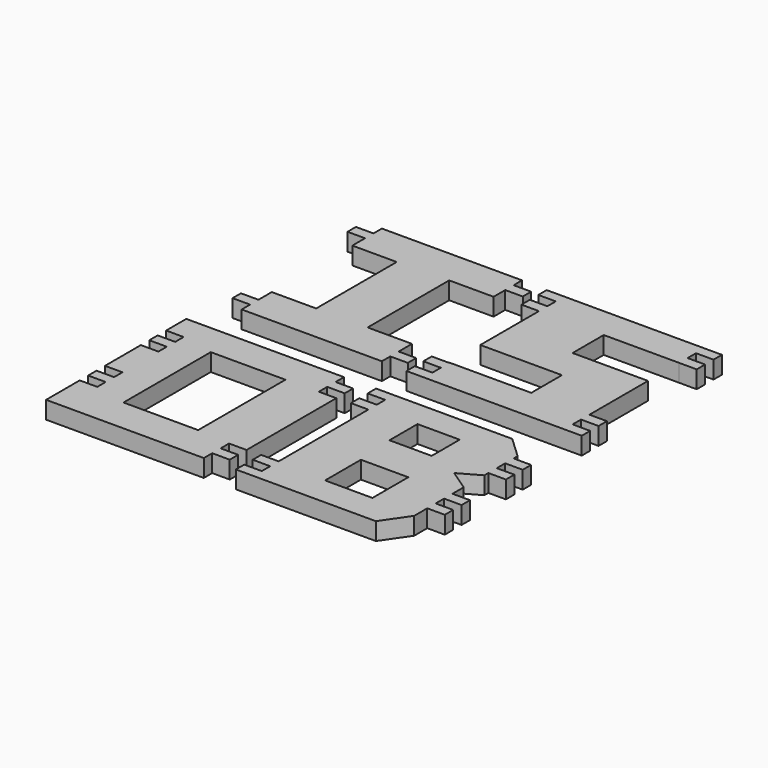
from build123d import *

# Parameters (mm, degrees)
F0_W     = 6.35
F0_H     = 3.81
F4_DEPTH = 6.35
F3_W     = 17.177414149
F3_H     = 16.2361897528
F3_W_2   = 15.2949504554
F3_H_2   = 12.7065815032
F3_W_3   = 6.35
F3_H_3   = 3.81
F5_DEPTH = 6.35
F1_W     = 6.35
F1_H     = 3.81
F6_DEPTH = 6.35
F2_W     = 27.0603150129
F2_H     = 39.5315941423
F7_DEPTH = 6.35


# Not quite as in the source:
# - a feature names something its author has since deleted; it is built from what else it names


with BuildPart() as f4:
    # F0 (on Top) → F4 (new body)
    with BuildSketch(Plane.XY):
        Polygon((57.15, 71.7689129657), (6.35, 71.7689129657), (6.35, 67.9589129657), (6.35, 64.1489129657), (6.35, 60.3389129657), (6.35, 33.7630063295), (35.9322190344, 33.7630063295), (35.9322190344, 19.8798868805), (6.35, 19.8798868805), (6.35, 19.6989129657), (6.35, 15.8889129657), (6.35, 12.0789129657), (6.35, 8.2689129657), (57.15, 8.2689129657), (57.15, 12.0789129657), (57.15, 15.8889129657), (57.15, 19.6989129657), (57.15, 46.2342835963), (29.8142325193, 46.2342835963), (29.8142325193, 60.3527091444), (57.15, 60.3527091444), (57.15, 64.1489129657), (57.15, 67.9589129657), align=None)
        with Locations((3.175, 69.8639129657)):
            Rectangle(F0_W, F0_H)
        with Locations((3.175, 62.2439129657)):
            Rectangle(F0_W, F0_H)
        with Locations((3.175, 17.7939129657)):
            Rectangle(F0_W, F0_H)
        with Locations((3.175, 10.1739129657)):
            Rectangle(F0_W, F0_H)
        with Locations((60.325, 69.8639129657)):
            Rectangle(F0_W, F0_H)
        Polygon((63.499985013, 64.1489129657), (57.15, 64.1489129657), (57.15, 60.3527091444), (63.499985013, 60.3389129657), align=None)
        with Locations((60.325, 17.7939129657)):
            Rectangle(F0_W, F0_H)
        with Locations((60.325, 10.1739129657)):
            Rectangle(F0_W, F0_H)
    extrude(amount=F4_DEPTH)


with BuildPart() as f5:
    # F3 (on Top) → F5 (new body)
    with BuildSketch(Plane.XY):
        Polygon((49.34674353, -5.4983740449), (6.35, -5.4983740449), (6.35, -9.3083740449), (6.35, -13.1183740449), (6.35, -16.9283740449), (6.35, -57.5683740449), (6.35, -61.3783740449), (6.35, -65.1883740449), (6.35, -68.9983740449), (50.7249496877, -68.9983740449), (57.15, -59.6539080143), (57.15, -53.7583740449), (57.15, -49.9483740449), (57.15, -46.1383740449), (57.15, -42.3283740449), (57.15, -37.2483740449), (49.582055217, -32.122977078), (57.15, -27.8874486685), (57.15, -26.0723740449), (57.15, -22.2623740449), (57.15, -18.4523740449), (57.15, -14.6423740449), (57.15, -12.8277968615), align=None)
        with Locations((32.488649711, -50.3592770547)):
            Rectangle(F3_W, F3_H, mode=Mode.SUBTRACT)
        with Locations((30.4045233935, -21.5341579169)):
            Rectangle(F3_W_2, F3_H_2, mode=Mode.SUBTRACT)
        with Locations((3.175, -7.4033740449)):
            Rectangle(F3_W_3, F3_H_3)
        with Locations((3.175, -15.0233740449)):
            Rectangle(F3_W_3, F3_H_3)
        with Locations((3.175, -59.4733740449)):
            Rectangle(F3_W_3, F3_H_3)
        with Locations((3.175, -67.0933740449)):
            Rectangle(F3_W_3, F3_H_3)
        with Locations((60.325, -16.5473740449)):
            Rectangle(F3_W_3, F3_H_3)
        with Locations((60.325, -24.1673740449)):
            Rectangle(F3_W_3, F3_H_3)
        with Locations((60.325, -44.2333740449)):
            Rectangle(F3_W_3, F3_H_3)
        with Locations((60.325, -51.8533740449)):
            Rectangle(F3_W_3, F3_H_3)
    extrude(amount=F5_DEPTH)


with BuildPart() as f6:
    # F1 (on Top) → F6 (new body)
    with BuildSketch(Plane.XY):
        with Locations((-63.1423869252, 66.3646499625)):
            Rectangle(F1_W, F1_H)
        Polygon((-9.1673869252, 72.0796499625), (-59.9673869252, 72.0796499625), (-59.9673869252, 68.2696499625), (-59.9673869252, 64.4596499625), (-59.9673869252, 60.6496499625), (-59.9673869252, 58.705560863), (-43.8845783249, 58.705560863), (-43.8845783249, 22.232959047), (-59.9673869252, 22.232959047), (-59.9673869252, 20.0096499625), (-59.9673869252, 16.1996499625), (-66.3173869252, 16.1996499625), (-66.3173869252, 12.3896499625), (-59.9673869252, 12.3896499625), (-59.9673869252, 8.5796499625), (-9.1673869252, 8.5796499625), (-9.1673869252, 12.3896499625), (-2.8173869252, 12.3896499625), (-2.8173869252, 16.1996499625), (-9.1673869252, 16.1996499625), (-9.1673869252, 20.0096499625), (-9.1673869252, 22.232959047), (-25.2501843252, 22.232959047), (-25.2501843252, 59.1761693358), (-9.1673869252, 59.1761693358), (-9.1673869252, 60.6496499625), (-9.1673869252, 64.4596499625), (-2.8173869252, 64.4596499625), (-2.8173869252, 68.2696499625), (-9.1673869252, 68.2696499625), align=None)
    extrude(amount=F6_DEPTH)


with BuildPart() as f7:
    # F2 (on Top) → F7 (new body)
    with BuildSketch(Plane.XY):
        Polygon((-11.4495668173, -5.7117735744), (-68.5995668173, -5.7117735744), (-68.5995668173, -14.8557735744), (-62.2495668173, -14.8557735744), (-62.2495668173, -18.6657735744), (-68.5995668173, -18.6657735744), (-68.5995668173, -22.4757735744), (-62.2495668173, -22.4757735744), (-62.2495668173, -26.2857735744), (-68.5995668173, -26.2857735744), (-68.5995668173, -42.5417735744), (-62.2495668173, -42.5417735744), (-62.2495668173, -46.3517735744), (-68.5995668173, -46.3517735744), (-68.5995668173, -50.1617735744), (-62.2495668173, -50.1617735744), (-62.2495668173, -53.9717735744), (-68.5995668173, -53.9717735744), (-68.5995668173, -69.2117735744), (-11.4495668173, -69.2117735744), (-11.4495668173, -65.4017735744), (-5.0995668173, -65.4017735744), (-5.0995668173, -61.5917735744), (-11.4495668173, -61.5917735744), (-11.4495668173, -57.7817735744), (-5.0995668173, -57.7817735744), (-5.0995668173, -17.1417735744), (-11.4495668173, -17.1417735744), (-11.4495668173, -13.3317735744), (-5.0995668173, -13.3317735744), (-5.0995668173, -9.5217735744), (-11.4495668173, -9.5217735744), align=None)
        with Locations((-36.9269400835, -37.0644265786)):
            Rectangle(F2_W, F2_H, mode=Mode.SUBTRACT)
    extrude(amount=F7_DEPTH)


solid = Compound([f4.part, f5.part, f6.part, f7.part])
